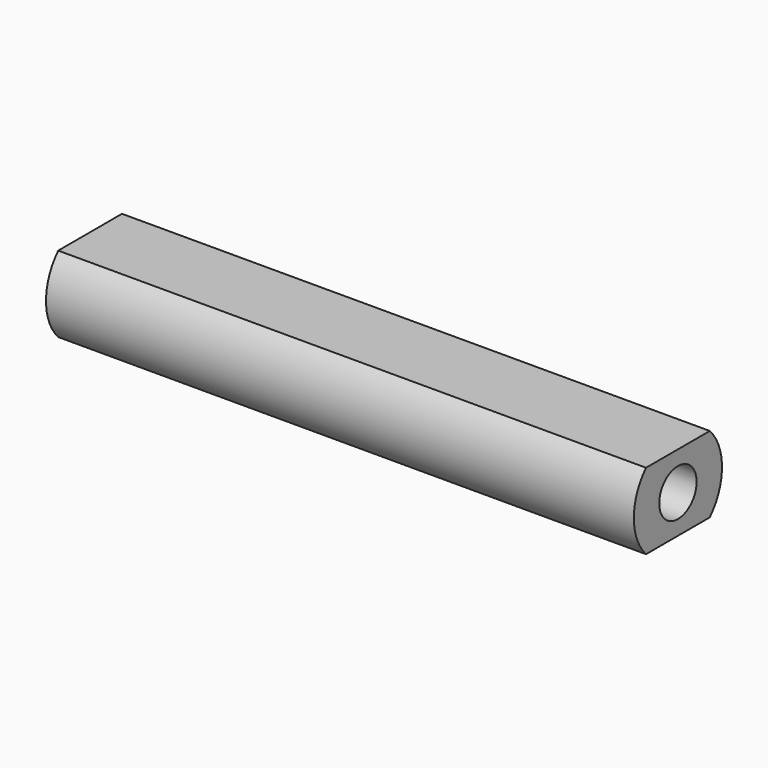
from build123d import *

# Parameters (mm, degrees)
F0_R     = 4.7625
F1_DEPTH = 50.8
F3_DEPTH = 50.801
F4_R     = 2.0193
F5_DEPTH = 44.45


# Not quite as in the source:
# - a pattern or mirror of a feature is missing from the dataset's text; its kind, count and spacing are read off the source's solid


with BuildPart() as f1:
    # F0 (on Right) → F1 (new body)
    with BuildSketch(Plane.YZ):
        Circle(F0_R)
    extrude(amount=F1_DEPTH)

    # F2 (on face) → F3 (cut, through all)
    with BuildSketch(Plane.YZ.offset(50.8)):
        with BuildLine():
            Line((-3.444112623, 3.2893), (3.444112623, 3.2893))
            ThreePointArc((3.444112623, 3.2893), (0, 4.7625), (-3.444112623, 3.2893))
        make_face()
    f3 = extrude(amount=-F3_DEPTH, mode=Mode.SUBTRACT)

    # F3_copies: F3 across plane
    add(f3.mirror(Plane(origin=(0, 0, 0), x_dir=(-1, 0, 0), z_dir=(0, 0, -1))), mode=Mode.SUBTRACT)

    # F4 (on face) → F5 (cut)
    with BuildSketch(Plane.YZ.offset(50.8)):
        Circle(F4_R)
    extrude(amount=-F5_DEPTH, mode=Mode.SUBTRACT)


solid = f1.part
